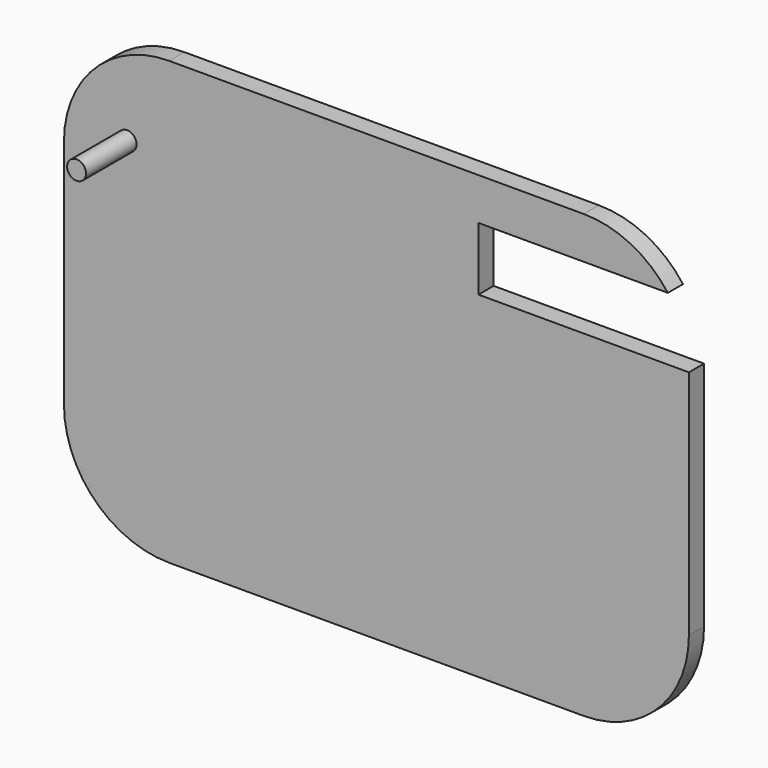
from build123d import *

# Parameters (mm, degrees)
F1_DEPTH = 9
F2_R     = 4.5
F3_DEPTH = 30
F5_W     = 100
F5_H     = 30
F6_DEPTH = 25


# Not quite as in the source:
# - the program builds the solid bodies; features that only make, move or delete a surface that nothing else refers to are left out


with BuildPart() as f1:
    # F0 (on Front) → F1 (new body)
    with BuildSketch(Plane.XZ):
        with BuildLine():
            Line((112.4640594495, 109.3449960649), (-84.5359405505, 109.3449960649))
            ThreePointArc((-84.5359405505, 109.3449960649), (-119.8912796099, 94.7003351242), (-134.5359405505, 59.3449960649))
            Line((-134.5359405505, 59.3449960649), (-134.5359405505, -50.6550039351))
            ThreePointArc((-134.5359405505, -50.6550039351), (-119.8912796099, -86.0103429944), (-84.5359405505, -100.6550039351))
            Line((-84.5359405505, -100.6550039351), (112.4640594495, -100.6550039351))
            ThreePointArc((112.4640594495, -100.6550039351), (147.8193985088, -86.0103429944), (162.4640594495, -50.6550039351))
            Line((162.4640594495, -50.6550039351), (162.4640594495, 59.3449960649))
            ThreePointArc((162.4640594495, 59.3449960649), (147.8193985088, 94.7003351242), (112.4640594495, 109.3449960649))
        make_face()
    extrude(amount=F1_DEPTH)

    # F2 (on face) → F3 (join)
    with BuildSketch(Plane.XZ.offset(9)):
        with Locations((-104.5359405505, 69.3449960649)):
            Circle(F2_R)
    extrude(amount=F3_DEPTH)

    # F5 (on face) → F6 (cut)
    with BuildSketch(Plane.XZ.offset(9)):
        with Locations((112.4640594495, 74.3449960649)):
            Rectangle(F5_W, F5_H)
    extrude(amount=-F6_DEPTH, mode=Mode.SUBTRACT)


solid = f1.part
